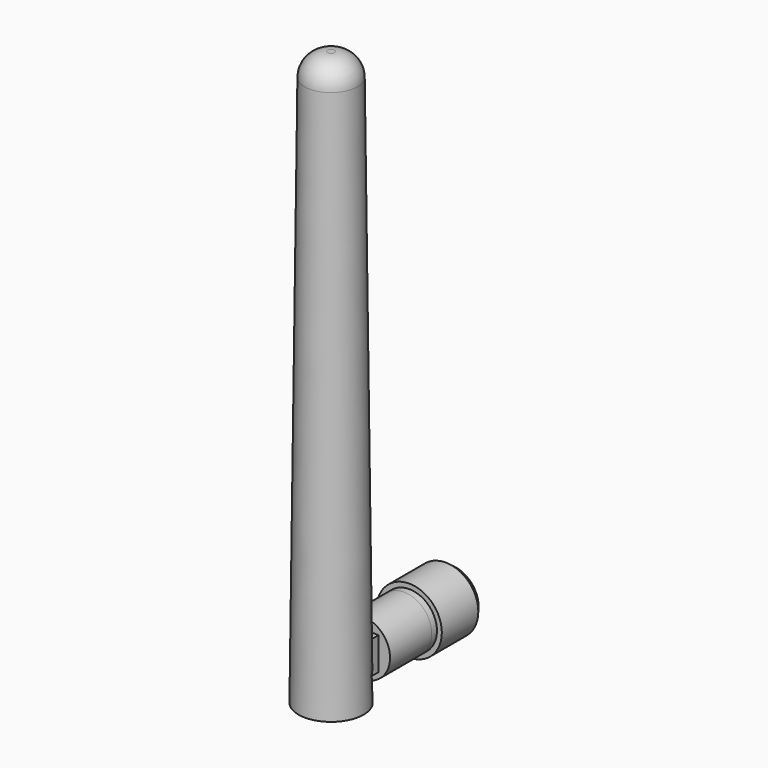
from build123d import *

# Parameters (mm, degrees)
F0_R     = 4.25
F1_DEPTH = 1
F2_R     = 5
F3_DEPTH = 7
F4_R     = 4.25
F5_DEPTH = 1
F6_DEPTH = 8
F7_W     = 5
F7_H     = 5
F8_DEPTH = 7
F9_R     = 2.49999
F11_R    = 5
F13_R    = 4
F15_R    = 3.5


# Not quite as in the source:
# - a fillet or chamfer is up to 0.001 mm smaller than in the source, because OpenCascade refuses the exact size


with BuildPart() as f1:
    # F0 (on Front) → F1 (new body)
    with BuildSketch(Plane.XZ):
        Circle(F0_R)
    extrude(amount=F1_DEPTH)

    # F2 (on face) → F3 (join)
    with BuildSketch(Plane.XZ.offset(1)):
        Circle(F2_R)
    extrude(amount=F3_DEPTH)

    # F4 (on face) → F5 (join)
    with BuildSketch(Plane.XZ.offset(8)):
        Circle(F4_R)
    extrude(amount=F5_DEPTH)


with BuildPart() as f6:
    # F6 (new): a face of the model
    f6_faces = [f1.part.faces().sort_by_distance(p)[0] for p in [
        (0, -9, 0),
    ]]
    extrude(f6_faces, amount=F6_DEPTH)

    # F7 (on face) → F8 (join)
    with BuildSketch(Plane.XZ.offset(17)):
        Rectangle(F7_W, F7_H)
    extrude(amount=F8_DEPTH)

    # F9 (radius 2.5 in the source; OpenCascade refuses exactly that, so slightly less here)
    f9_edges = [f6.edges().sort_by_distance(p)[0] for p in [
        (0, -24, 2.5),
        (0, -24, -2.5),
    ]]
    fillet(f9_edges, radius=F9_R)

    # F11 (on offset) → F14 section 0
    with BuildSketch(Plane.XY.offset(-5)):
        with Locations((0, -23)):
            Circle(F11_R)
    # F13 (on offset) → F14 section 1
    with BuildSketch(Plane.XY.offset(83)):
        with Locations((0, -23)):
            Circle(F13_R)
    loft()

    # F15
    f15_edges = [f6.edges().sort_by_distance(p)[0] for p in [
        (-4, -23, 83),
    ]]
    fillet(f15_edges, radius=F15_R)


solid = Compound([f1.part, f6.part])
